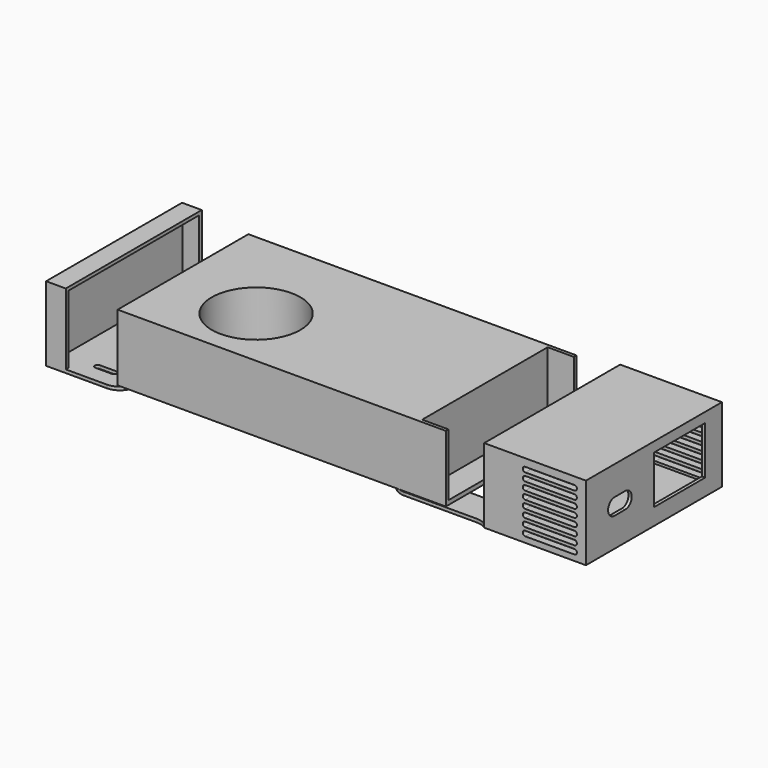
from build123d import *

# Parameters (mm, degrees)
F0_W          = 200
F0_H          = 99.6
F1_DEPTH      = 40.6
F2_W          = 16
F2_H          = 95.6
F2_R          = 27
F3_DEPTH      = 38
F4_R          = 1.6
F5_DEPTH      = 25
F7_W          = 103.6
F7_H          = 45.4
F7_W_2        = 94.8
F7_H_2        = 41.4
F8_DEPTH      = 60
F9_W          = 103.6
F9_H          = 45.4
F9_W_2        = 94.8
F9_H_2        = 41.4
F10_DEPTH     = 2
F11_W         = 39
F11_H         = 29.3
F12_DEPTH     = 2
F13_W         = 99.6
F13_H         = 41.4
F14_DEPTH     = 20
F15_W         = 19
F15_H         = 2
F16_DEPTH     = 60
F17_T1_DEPTH  = 2
F17_T3_DEPTH  = 2
F17_T5_DEPTH  = 2
F17_T7_DEPTH  = 2
F17_T9_DEPTH  = 49.5
F17_T11_DEPTH = 49.5
F17_T13_DEPTH = 49.5
F17_T15_DEPTH = 49.5
F19_DEPTH     = 2.401
F21_DEPTH     = 103.601
F23_W         = 103.6
F23_H         = 45.4
F23_W_2       = 99.6
F23_H_2       = 41.4
F24_DEPTH     = 10
F25_W         = 103.6
F25_H         = 45.4
F26_DEPTH     = 2
F27_W         = 103.6
F27_H         = 2
F28_DEPTH     = 35
F29_R         = 10
F31_DEPTH     = 2


# Not quite as in the source:
# - a fillet or chamfer that OpenCascade refuses, or shapes differently, is made with other operations: its cross-section is extruded or revolved along the edge and cut away or added


with BuildPart() as f1:
    # F0 (on Top) → F1 (new body)
    with BuildSketch(Plane.XY):
        Rectangle(F0_W, F0_H)
    extrude(amount=F1_DEPTH)

    # F2 (on face) → F3 (cut)
    with BuildSketch(Plane.XY.offset(40.6)):
        with Locations((92, 0)):
            Rectangle(F2_W, F2_H)
        with Locations((-46, -11.8)):
            Circle(F2_R)
    extrude(amount=-F3_DEPTH, mode=Mode.SUBTRACT)

    # F4 (on face) → F5 (cut)
    with BuildSketch(Plane(origin=(0, 0, 0), x_dir=(1, 0, 0), z_dir=(0, 0, -1))):
        with Locations((-75, 25)):
            Circle(F4_R)
        with Locations((75, 25)):
            Circle(F4_R)
        with Locations((-75, -25)):
            Circle(F4_R)
        with Locations((75, -25)):
            Circle(F4_R)
    extrude(amount=-F5_DEPTH, mode=Mode.SUBTRACT)


with BuildPart() as f8:
    # F7 (on offset) → F8 (new body)
    with BuildSketch(Plane.YZ.offset(125)):
        with Locations((0, 20.3)):
            Rectangle(F7_W, F7_H)
        with Locations((0, 20.3)):
            Rectangle(F7_W_2, F7_H_2, mode=Mode.SUBTRACT)
    extrude(amount=F8_DEPTH)

    # F9 (on face) → F10 (join)
    with BuildSketch(Plane.YZ.offset(185)):
        with Locations((0, 20.3)):
            Rectangle(F9_W, F9_H)
        with Locations((0, 20.3)):
            Rectangle(F9_W_2, F9_H_2, mode=Mode.SUBTRACT)
        with Locations((0, 20.3)):
            Rectangle(F9_W_2, F9_H_2)
    extrude(amount=F10_DEPTH)

    # F11 (on face) → F12 (cut, through all)
    with BuildSketch(Plane.YZ.offset(187)):
        with Locations((19.5, 22.35)):
            Rectangle(F11_W, F11_H)
        with BuildLine():
            ThreePointArc((-29.9, 25.3), (-34.9, 20.3), (-29.9, 15.3))
            Line((-29.9, 15.3), (-21.9, 15.3))
            ThreePointArc((-21.9, 15.3), (-16.9, 20.3), (-21.9, 25.3))
            Line((-21.9, 25.3), (-29.9, 25.3))
        make_face()
    extrude(amount=-F12_DEPTH, mode=Mode.SUBTRACT)

    # F13 (on face) → F14 (cut)
    with BuildSketch(Plane(origin=(125, 0, 0), x_dir=(0, -1, 0), z_dir=(-1, 0, 0))):
        with Locations((0, 20.3)):
            Rectangle(F13_W, F13_H)
    extrude(amount=-F14_DEPTH, mode=Mode.SUBTRACT)

    # F15 (on face) → F16 (join)
    with BuildSketch(Plane(origin=(125, 0, 0), x_dir=(0, -1, 0), z_dir=(-1, 0, 0))):
        with Locations((-40.3, -1.4)):
            Rectangle(F15_W, F15_H)
        with Locations((40.3, -1.4)):
            Rectangle(F15_W, F15_H)
    extrude(amount=F16_DEPTH)

    # F17: fillet of radius 9.5 on 8 edges, made by hand

    # F17_s2 → F17_t1 (join)
    with BuildSketch(Plane.XY.offset(-2.4)):
        with BuildLine():
            ThreePointArc((125, 51.8), (122.2512551066, 50.3138996222), (119.1690481052, 49.8))
            Line((119.1690481052, 49.8), (125, 49.8))
            Line((125, 49.8), (125, 51.8))
        make_face()
    extrude(amount=F17_T1_DEPTH)

    # F17_s4 → F17_t3 (join)
    with BuildSketch(Plane.XY.offset(-2.4)):
        with BuildLine():
            ThreePointArc((125, -51.8), (122.2512551066, -50.3138996222), (119.1690481052, -49.8))
            Line((119.1690481052, -49.8), (125, -49.8))
            Line((125, -49.8), (125, -51.8))
        make_face()
    extrude(amount=F17_T3_DEPTH)

    # F17_s6 → F17_t5 (join)
    with BuildSketch(Plane.XY.offset(-2.4)):
        with BuildLine():
            ThreePointArc((125, -21.3), (122.2175144213, -28.0175144213), (115.5, -30.8))
            Line((115.5, -30.8), (125, -30.8))
            Line((125, -30.8), (125, -21.3))
        make_face()
    extrude(amount=F17_T5_DEPTH)

    # F17_s8 → F17_t7 (join)
    with BuildSketch(Plane.XY.offset(-2.4)):
        with BuildLine():
            ThreePointArc((115.5, 30.8), (122.2175144213, 28.0175144213), (125, 21.3))
            Line((125, 21.3), (125, 30.8))
            Line((125, 30.8), (115.5, 30.8))
        make_face()
    extrude(amount=F17_T7_DEPTH)

    # F17_s10 → F17_t9 (cut)
    with BuildSketch(Plane.XY.offset(-26.15)):
        with BuildLine():
            ThreePointArc((74.5, 49.8), (67.7824855787, 47.0175144213), (65, 40.3))
            Line((65, 40.3), (65, 49.8))
            Line((65, 49.8), (74.5, 49.8))
        make_face()
    extrude(amount=F17_T9_DEPTH, mode=Mode.SUBTRACT)

    # F17_s12 → F17_t11 (cut)
    with BuildSketch(Plane.XY.offset(-26.15)):
        with BuildLine():
            ThreePointArc((74.5, -49.8), (67.7824855787, -47.0175144213), (65, -40.3))
            Line((65, -40.3), (65, -49.8))
            Line((65, -49.8), (74.5, -49.8))
        make_face()
    extrude(amount=F17_T11_DEPTH, mode=Mode.SUBTRACT)

    # F17_s14 → F17_t13 (cut)
    with BuildSketch(Plane.XY.offset(-26.15)):
        with BuildLine():
            ThreePointArc((65, -40.3), (67.7824855787, -33.5824855787), (74.5, -30.8))
            Line((74.5, -30.8), (65, -30.8))
            Line((65, -30.8), (65, -40.3))
        make_face()
    extrude(amount=F17_T13_DEPTH, mode=Mode.SUBTRACT)

    # F17_s16 → F17_t15 (cut)
    with BuildSketch(Plane.XY.offset(-26.15)):
        with BuildLine():
            ThreePointArc((74.5, 30.8), (67.7824855787, 33.5824855787), (65, 40.3))
            Line((65, 40.3), (65, 30.8))
            Line((65, 30.8), (74.5, 30.8))
        make_face()
    extrude(amount=F17_T15_DEPTH, mode=Mode.SUBTRACT)

    # F18 (on face) → F19 (cut, through all)
    with BuildSketch(Plane(origin=(0, 0, 0), x_dir=(1, 0, 0), z_dir=(0, 0, -1))):
        with BuildLine():
            ThreePointArc((80, 41.7), (78.3, 40), (80, 38.3))
            Line((80, 38.3), (90, 38.3))
            ThreePointArc((90, 38.3), (91.7, 40), (90, 41.7))
            Line((90, 41.7), (80, 41.7))
        make_face()
        with BuildLine():
            Line((90, -38.3), (80, -38.3))
            ThreePointArc((80, -38.3), (78.3, -40), (80, -41.7))
            Line((80, -41.7), (90, -41.7))
            ThreePointArc((90, -41.7), (91.7, -40), (90, -38.3))
        make_face()
    extrude(amount=F19_DEPTH, mode=Mode.SUBTRACT)

    # F20 (on face) → F21 (cut, through all)
    with BuildSketch(Plane.XZ.offset(51.8)):
        with BuildLine():
            ThreePointArc((150, 4.1), (148.5, 2.6), (150, 1.1))
            Line((150, 1.1), (180, 1.1))
            ThreePointArc((180, 1.1), (181.5, 2.6), (180, 4.1))
            Line((180, 4.1), (150, 4.1))
        make_face()
        with BuildLine():
            ThreePointArc((150, 9), (148.5, 7.5), (150, 6))
            Line((150, 6), (180, 6))
            ThreePointArc((180, 6), (181.5, 7.5), (180, 9))
            Line((180, 9), (150, 9))
        make_face()
        with BuildLine():
            ThreePointArc((150, 13.9), (148.5, 12.4), (150, 10.9))
            Line((150, 10.9), (180, 10.9))
            ThreePointArc((180, 10.9), (181.5, 12.4), (180, 13.9))
            Line((180, 13.9), (150, 13.9))
        make_face()
        with BuildLine():
            ThreePointArc((150, 18.8), (148.5, 17.3), (150, 15.8))
            Line((150, 15.8), (180, 15.8))
            ThreePointArc((180, 15.8), (181.5, 17.3), (180, 18.8))
            Line((180, 18.8), (150, 18.8))
        make_face()
        with BuildLine():
            ThreePointArc((150, 23.7), (148.5, 22.2), (150, 20.7))
            Line((150, 20.7), (180, 20.7))
            ThreePointArc((180, 20.7), (181.5, 22.2), (180, 23.7))
            Line((180, 23.7), (150, 23.7))
        make_face()
        with BuildLine():
            ThreePointArc((150, 28.6), (148.5, 27.1), (150, 25.6))
            Line((150, 25.6), (180, 25.6))
            ThreePointArc((180, 25.6), (181.5, 27.1), (180, 28.6))
            Line((180, 28.6), (150, 28.6))
        make_face()
        with BuildLine():
            ThreePointArc((150, 33.5), (148.5, 32), (150, 30.5))
            Line((150, 30.5), (180, 30.5))
            ThreePointArc((180, 30.5), (181.5, 32), (180, 33.5))
            Line((180, 33.5), (150, 33.5))
        make_face()
        with BuildLine():
            ThreePointArc((150, 38.4), (148.5, 36.9), (150, 35.4))
            Line((150, 35.4), (180, 35.4))
            ThreePointArc((180, 35.4), (181.5, 36.9), (180, 38.4))
            Line((180, 38.4), (150, 38.4))
        make_face()
    extrude(amount=-F21_DEPTH, mode=Mode.SUBTRACT)


with BuildPart() as f24:
    # F23 (on offset) → F24 (new body)
    with BuildSketch(Plane(origin=(-140, 0, 0), x_dir=(0, -1, 0), z_dir=(-1, 0, 0))):
        with Locations((0, 20.3)):
            Rectangle(F23_W, F23_H)
        with Locations((0, 20.3)):
            Rectangle(F23_W_2, F23_H_2, mode=Mode.SUBTRACT)
    extrude(amount=-F24_DEPTH)

    # F25 (on face) → F26 (join)
    with BuildSketch(Plane(origin=(-140, 0, 0), x_dir=(0, -1, 0), z_dir=(-1, 0, 0))):
        with Locations((0, 20.3)):
            Rectangle(F25_W, F25_H)
    extrude(amount=F26_DEPTH)

    # F27 (on face) → F28 (join)
    with BuildSketch(Plane.YZ.offset(-130)):
        with Locations((0, -1.4)):
            Rectangle(F27_W, F27_H)
    extrude(amount=F28_DEPTH)

    # F29
    f29_edges = [f24.edges().sort_by_distance(p)[0] for p in [
        (-95, -51.8, -1.4),
        (-95, 51.8, -1.4),
    ]]
    fillet(f29_edges, radius=F29_R)

    # F30 (on face) → F31 (cut, through all)
    with BuildSketch(Plane(origin=(0, 0, -2.4), x_dir=(1, 0, 0), z_dir=(0, 0, -1))):
        with BuildLine():
            ThreePointArc((-120, 41.7), (-121.7, 40), (-120, 38.3))
            Line((-120, 38.3), (-110, 38.3))
            ThreePointArc((-110, 38.3), (-108.3, 40), (-110, 41.7))
            Line((-110, 41.7), (-120, 41.7))
        make_face()
        with BuildLine():
            Line((-110, -38.3), (-120, -38.3))
            ThreePointArc((-120, -38.3), (-121.7, -40), (-120, -41.7))
            Line((-120, -41.7), (-110, -41.7))
            ThreePointArc((-110, -41.7), (-108.3, -40), (-110, -38.3))
        make_face()
    extrude(amount=-F31_DEPTH, mode=Mode.SUBTRACT)


solid = Compound([f1.part, f8.part, f24.part])
